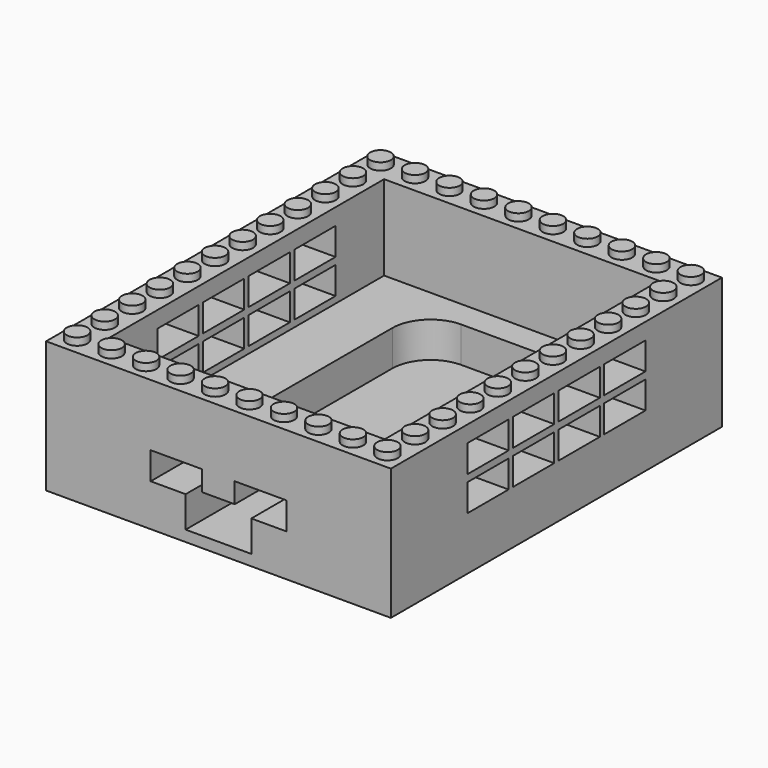
from build123d import *

# Parameters (mm, degrees)
F0_W      = 80
F0_H      = 96
F0_W_2    = 63.8302
F0_H_2    = 79.6163
F1_DEPTH  = 27.94
F2_W      = 80
F2_H      = 96
F2_W_2    = 63.8302
F2_H_2    = 79.6163
F3_DEPTH  = 2.54
F4_W      = 63.8302
F4_H      = 79.6163
F5_DEPTH  = 8.255
F6_W      = 7.62
F6_H      = 8.89
F7_DEPTH  = 25.4
F9_DEPTH  = 19.05
F10_W     = 11.9634
F10_H     = 6.35
F11_DEPTH = 127
F12_R     = 2.4
F13_DEPTH = 1.7


# Not quite as in the source:
# - a feature names something its author has since deleted; it is built from what else it names


with BuildPart() as f1:
    # F0 (on Top) → F1 (new body)
    with BuildSketch(Plane.XY):
        with Locations((31.9151, -39.9151)):
            Rectangle(F0_W, F0_H)
        with Locations((31.9151, -39.80815)):
            Rectangle(F0_W_2, F0_H_2, mode=Mode.SUBTRACT)
    extrude(amount=F1_DEPTH)

    # F2 (on Top) → F3 (join)
    with BuildSketch(Plane.XY):
        with Locations((31.9151, -39.9151)):
            Rectangle(F2_W, F2_H)
        with Locations((31.9151, -39.80815)):
            Rectangle(F2_W_2, F2_H_2, mode=Mode.SUBTRACT)
        with Locations((31.9151, -39.80815)):
            Rectangle(F2_W_2, F2_H_2)
    extrude(amount=-F3_DEPTH)

    # F4 (on face) → F5 (join)
    with BuildSketch(Plane.XY):
        with Locations((31.9151, -39.80815)):
            Rectangle(F4_W, F4_H)
        with BuildLine():
            ThreePointArc((14.01445, -15.14475), (16.6182707153, -8.8585707153), (22.90445, -6.25475))
            Line((22.90445, -6.25475), (40.93845, -6.25475))
            ThreePointArc((40.93845, -6.25475), (47.2246292847, -8.8585707153), (49.82845, -15.14475))
            Line((49.82845, -15.14475), (49.82845, -63.40475))
            ThreePointArc((49.82845, -63.40475), (47.2246292847, -69.6909292847), (40.93845, -72.29475))
            Line((40.93845, -72.29475), (35.73145, -72.29475))
            Line((35.73145, -72.29475), (35.73145, -73.81875))
            Line((35.73145, -73.81875), (32.30245, -73.81875))
            Line((32.30245, -73.81875), (31.92145, -73.81875))
            Line((31.92145, -73.81875), (28.11145, -73.81875))
            Line((28.11145, -73.81875), (28.11145, -72.29475))
            Line((28.11145, -72.29475), (22.90445, -72.29475))
            ThreePointArc((22.90445, -72.29475), (16.6182707153, -69.6909292847), (14.01445, -63.40475))
            Line((14.01445, -63.40475), (14.01445, -15.14475))
        make_face(mode=Mode.SUBTRACT)
    extrude(amount=F5_DEPTH)

    # F6 (on face) → F7 (cut)
    with BuildSketch(Plane.XZ.offset(87.9151)):
        Polygon((39.5351, 8.89), (31.9151, 8.89), (31.9151, 0), (36.9951, 0), (39.5351, 0), align=None)
        with Locations((28.1051, 4.445)):
            Rectangle(F6_W, F6_H)
    extrude(amount=-F7_DEPTH, mode=Mode.SUBTRACT)

    # F8 (on face) → F9 (cut)
    with BuildSketch(Plane.XZ.offset(87.9151)):
        Polygon((28.1432, 13.589), (16.1798, 13.589), (16.1798, 7.239), (24.2951, 7.239), (24.2951, 8.89), (28.1432, 8.89), align=None)
        Polygon((35.687, 13.589), (35.687, 8.89), (39.5351, 8.89), (39.5351, 7.239), (47.6504, 7.239), (47.6504, 13.589), align=None)
    extrude(amount=-F9_DEPTH, mode=Mode.SUBTRACT)

    # F10 (on face) → F11 (cut)
    with BuildSketch(Plane.YZ.offset(71.9151)):
        with Locations((-33.2984, 20.955)):
            Rectangle(F10_W, F10_H)
        with Locations((-20.065, 20.955)):
            Rectangle(F10_W, F10_H)
        with Locations((-46.5318, 20.955)):
            Rectangle(F10_W, F10_H)
        with Locations((-59.7652, 20.955)):
            Rectangle(F10_W, F10_H)
        with Locations((-20.065, 12.9794)):
            Rectangle(F10_W, F10_H)
        with Locations((-33.2984, 12.9794)):
            Rectangle(F10_W, F10_H)
        with Locations((-46.5318, 12.9794)):
            Rectangle(F10_W, F10_H)
        with Locations((-59.7652, 12.9794)):
            Rectangle(F10_W, F10_H)
    extrude(amount=-F11_DEPTH, mode=Mode.SUBTRACT)

    # F12 (on face) → F13 (join)
    with BuildSketch(Plane.XY.offset(27.94)):
        with Locations((-4.0849, -83.9151)):
            Circle(F12_R)
        with Locations((3.9151, -83.9151)):
            Circle(F12_R)
        with Locations((11.9151, -83.9151)):
            Circle(F12_R)
        with Locations((19.9151, -83.9151)):
            Circle(F12_R)
        with Locations((27.9151, -83.9151)):
            Circle(F12_R)
        with Locations((35.9151, -83.9151)):
            Circle(F12_R)
        with Locations((43.9151, -83.9151)):
            Circle(F12_R)
        with Locations((51.9151, -83.9151)):
            Circle(F12_R)
        with Locations((67.9151, -83.9151)):
            Circle(F12_R)
        with Locations((59.9151, -83.9151)):
            Circle(F12_R)
        with Locations((67.9151, -75.9151)):
            Circle(F12_R)
        with Locations((67.9151, -67.9151)):
            Circle(F12_R)
        with Locations((67.9151, -59.9151)):
            Circle(F12_R)
        with Locations((67.9151, -51.9151)):
            Circle(F12_R)
        with Locations((67.9151, -43.9151)):
            Circle(F12_R)
        with Locations((67.9151, -35.9151)):
            Circle(F12_R)
        with Locations((67.9151, -27.9151)):
            Circle(F12_R)
        with Locations((67.9151, -19.9151)):
            Circle(F12_R)
        with Locations((67.9151, -11.9151)):
            Circle(F12_R)
        with Locations((67.9151, -3.9151)):
            Circle(F12_R)
        with Locations((-4.0849, -75.9151)):
            Circle(F12_R)
        with Locations((-4.0849, -67.9151)):
            Circle(F12_R)
        with Locations((-4.0849, -59.9151)):
            Circle(F12_R)
        with Locations((-4.0849, -51.9151)):
            Circle(F12_R)
        with Locations((-4.0849, -43.9151)):
            Circle(F12_R)
        with Locations((-4.0849, -35.9151)):
            Circle(F12_R)
        with Locations((-4.0849, -27.9151)):
            Circle(F12_R)
        with Locations((-4.0849, -19.9151)):
            Circle(F12_R)
        with Locations((-4.0849, -11.9151)):
            Circle(F12_R)
        with Locations((-4.0849, -3.9151)):
            Circle(F12_R)
        with Locations((-4.0849, 4.0849)):
            Circle(F12_R)
        with Locations((3.9151, 4.0849)):
            Circle(F12_R)
        with Locations((11.9151, 4.0849)):
            Circle(F12_R)
        with Locations((19.9151, 4.0849)):
            Circle(F12_R)
        with Locations((27.9151, 4.0849)):
            Circle(F12_R)
        with Locations((59.9151, 4.0849)):
            Circle(F12_R)
        with Locations((51.9151, 4.0849)):
            Circle(F12_R)
        with Locations((43.9151, 4.0849)):
            Circle(F12_R)
        with Locations((35.9151, 4.0849)):
            Circle(F12_R)
        with Locations((67.9151, 4.0849)):
            Circle(F12_R)
    extrude(amount=F13_DEPTH)


solid = f1.part
